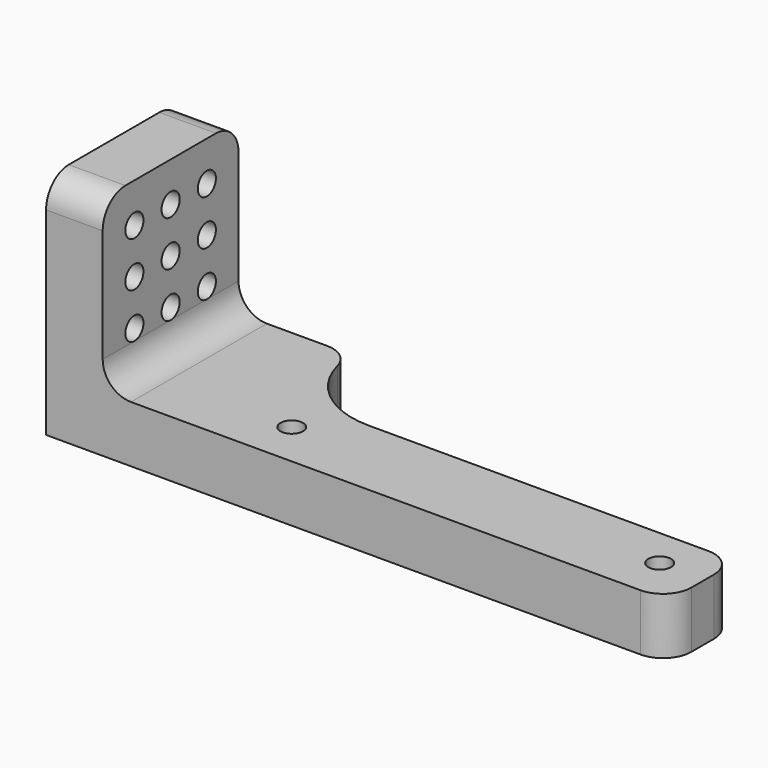
from build123d import *

# Parameters (mm, degrees)
F0_W     = 110
F0_H     = 30
F1_DEPTH = 10
F2_R     = 2
F3_DEPTH = 25
F4_W     = 10
F4_H     = 30
F5_DEPTH = 30
F6_R     = 2
F7_DEPTH = 25
F8_R     = 4.99999


# Not quite as in the source:
# - a fillet or chamfer is up to 0.001 mm smaller than in the source, because OpenCascade refuses the exact size
# - a feature names something its author has since deleted; it is built from what else it names


with BuildPart() as f1:
    # F0 (on Top) → F1 (new body)
    with BuildSketch(Plane.XY):
        with Locations((-55, 15)):
            Rectangle(F0_W, F0_H)
    extrude(amount=F1_DEPTH)

    # F2 (on face) → F3 (cut)
    with BuildSketch(Plane(origin=(0, 0, 0), x_dir=(1, 0, 0), z_dir=(0, 0, -1))):
        with Locations((-8, -8)):
            Circle(F2_R)
        with Locations((-73, -8)):
            Circle(F2_R)
        with BuildLine():
            Line((0, -30), (0, -15))
            Line((0, -15), (-65, -15))
            ThreePointArc((-65, -15), (-75.6066017178, -19.3933982822), (-80, -30))
            Line((-80, -30), (0, -30))
        make_face()
    extrude(amount=-F3_DEPTH, mode=Mode.SUBTRACT)

    # F4 (on face) → F5 (join)
    with BuildSketch(Plane.XY.offset(10)):
        with Locations((-105, 15)):
            Rectangle(F4_W, F4_H)
    extrude(amount=F5_DEPTH)

    # F6 (on face) → F7 (cut)
    with BuildSketch(Plane.YZ.offset(-100)):
        with Locations((7, 17)):
            Circle(F6_R)
        with Locations((7, 25)):
            Circle(F6_R)
        with Locations((15, 33)):
            Circle(F6_R)
        with Locations((7, 33)):
            Circle(F6_R)
        with Locations((15, 25)):
            Circle(F6_R)
        with Locations((15, 17)):
            Circle(F6_R)
        with Locations((23, 17)):
            Circle(F6_R)
        with Locations((23, 25)):
            Circle(F6_R)
        with Locations((23, 33)):
            Circle(F6_R)
    extrude(amount=-F7_DEPTH, mode=Mode.SUBTRACT)

    # F8 (radius 5 in the source; OpenCascade refuses exactly that, so slightly less here)
    f8_edges = [f1.edges().sort_by_distance(p)[0] for p in [
        (0, 15, 5),
        (0, 0, 5),
        (-80, 30, 5),
        (-105, 30, 40),
        (-105, 0, 40),
        (-100, 15, 10),
    ]]
    fillet(f8_edges, radius=F8_R)


solid = f1.part
